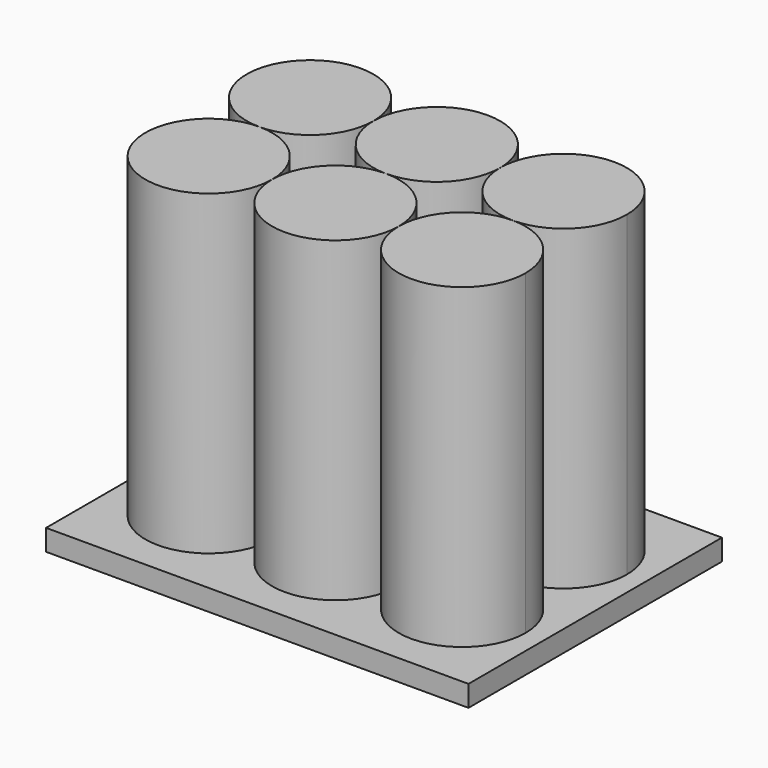
from build123d import *

# Parameters (mm, degrees)
F1_DEPTH = 76.2
F2_W     = 101.6
F2_H     = 5.08
F3_DEPTH = 38.1


# Not quite as in the source:
# - a feature names something its author has since deleted; it is built from what else it names


with BuildPart() as f1:
    # F0 (on Top) → F1 (new body)
    with BuildSketch(Plane.XY):
        with BuildLine():
            ThreePointArc((-29.9686177893, -0.0085821988), (-40.7449251346, -26.0248895441), (-14.7286177893, -15.2485821988))
            ThreePointArc((-14.7286177893, -15.2485821988), (-19.192310444, -4.4722748535), (-29.9686177893, -0.0085821988))
        make_face()
    extrude(amount=F1_DEPTH)


with BuildPart() as f1b:
    # F0 (on Top) → F1, piece 2 (new body)
    with BuildSketch(Plane.XY):
        with BuildLine():
            ThreePointArc((0.5113822094, -0.0085821988), (-10.264925135, -4.472274854), (-14.7286177893, -15.2485821988))
            ThreePointArc((-14.7286177893, -15.2485821988), (0.5113822107, -30.4885821988), (15.7513822107, -15.2485821988))
            ThreePointArc((15.7513822107, -15.2485821988), (11.2876895555, -4.4722748531), (0.5113822094, -0.0085821988))
        make_face()
    extrude(amount=F1_DEPTH)


with BuildPart() as f1c:
    # F0 (on Top) → F1, piece 3 (new body)
    with BuildSketch(Plane.XY):
        with BuildLine():
            ThreePointArc((-14.7286177893, 15.2314178012), (-40.7449251346, 26.0077251465), (-29.9686177893, -0.0085821988))
            ThreePointArc((-29.9686177893, -0.0085821988), (-19.192310444, 4.4551104559), (-14.7286177893, 15.2314178012))
        make_face()
    extrude(amount=F1_DEPTH)


with BuildPart() as f1d:
    # F0 (on Top) → F1, piece 4 (new body)
    with BuildSketch(Plane.XY):
        with BuildLine():
            ThreePointArc((30.9913822354, -0.0085821988), (20.2150748742, -4.4722748448), (15.7513822107, -15.2485821988))
            ThreePointArc((15.7513822107, -15.2485821988), (30.9913822107, -30.4885821988), (46.2313822107, -15.2485821988))
            ThreePointArc((46.2313822107, -15.2485821988), (41.7676895647, -4.4722748623), (30.9913822354, -0.0085821988))
        make_face()
    extrude(amount=F1_DEPTH)


with BuildPart() as f1e:
    # F0 (on Top) → F1, piece 5 (new body)
    with BuildSketch(Plane.XY):
        with BuildLine():
            ThreePointArc((-14.7286177893, 15.2314178012), (-10.264925135, 4.4551104564), (0.5113822094, -0.0085821988))
            ThreePointArc((0.5113822094, -0.0085821988), (11.2876895555, 4.4551104555), (15.7513822107, 15.2314178012))
            ThreePointArc((15.7513822107, 15.2314178012), (0.5113822107, 30.4714178012), (-14.7286177893, 15.2314178012))
        make_face()
    extrude(amount=F1_DEPTH)


with BuildPart() as f1f:
    # F0 (on Top) → F1, piece 6 (new body)
    with BuildSketch(Plane.XY):
        with BuildLine():
            ThreePointArc((15.7513822107, 15.2314178012), (20.2150748742, 4.4551104472), (30.9913822354, -0.0085821988))
            ThreePointArc((30.9913822354, -0.0085821988), (41.7676895647, 4.4551104647), (46.2313822107, 15.2314178012))
            ThreePointArc((46.2313822107, 15.2314178012), (30.9913822107, 30.4714178012), (15.7513822107, 15.2314178012))
        make_face()
    extrude(amount=F1_DEPTH)


with BuildPart() as f3:
    # F2 (on Front) → F3 (new body, symmetric)
    with BuildSketch(Plane.XZ):
        with Locations((0, -2.54)):
            Rectangle(F2_W, F2_H)
    extrude(amount=F3_DEPTH, both=True)


solid = Compound([f1.part, f1b.part, f1c.part, f1d.part, f1e.part, f1f.part, f3.part])
